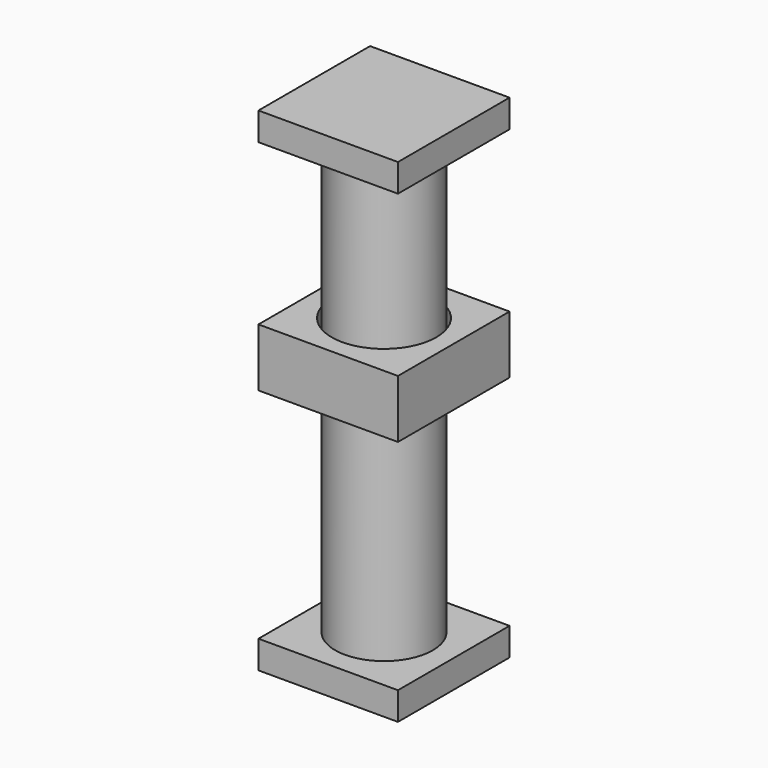
from build123d import *

# Parameters (mm, degrees)
F0_W     = 60
F0_H     = 60
F1_DEPTH = 25
F2_R     = 22.5
F3_DEPTH = 25
F4_R     = 21
F5_DEPTH = 100
F6_W     = 60
F6_H     = 60
F6_R     = 21
F7_DEPTH = 6
F8_W     = 60
F8_H     = 60
F8_R     = 21
F9_DEPTH = 6


with BuildPart() as f1:
    # F0 (on Top) → F1 (new body)
    with BuildSketch(Plane.XY):
        Rectangle(F0_W, F0_H)
    extrude(amount=F1_DEPTH)

    # F2 (on face) → F3 (cut)
    with BuildSketch(Plane.XY.offset(25)):
        Circle(F2_R)
    extrude(amount=-F3_DEPTH, mode=Mode.SUBTRACT)


with BuildPart() as f5:
    # F4 (on Top) → F5 (new body, symmetric)
    with BuildSketch(Plane.XY):
        Circle(F4_R)
    extrude(amount=F5_DEPTH, both=True)

    # F6 (on face) → F7 (join, symmetric)
    with BuildSketch(Plane.XY.offset(100)):
        Rectangle(F6_W, F6_H)
        Circle(F6_R, mode=Mode.SUBTRACT)
        Circle(F6_R)
    extrude(amount=F7_DEPTH, both=True)

    # F8 (on face) → F9 (join, symmetric)
    with BuildSketch(Plane(origin=(0, 0, -100), x_dir=(1, 0, 0), z_dir=(0, 0, -1))):
        Rectangle(F8_W, F8_H)
        Circle(F8_R, mode=Mode.SUBTRACT)
        Circle(F8_R)
    extrude(amount=F9_DEPTH, both=True)


solid = Compound([f1.part, f5.part])
